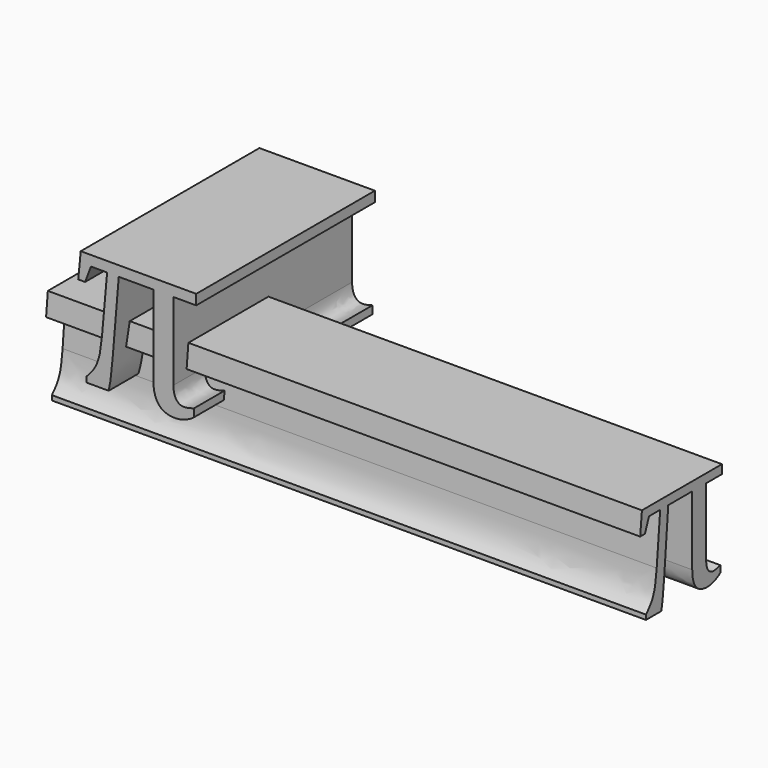
from build123d import *

# Parameters (mm, degrees)
F0_TEXT_SIZE = 28.1909998092
F1_DEPTH     = 25.4
F2_TEXT_SIZE = 24.4161502148
F3_DEPTH     = 67.564


# Not quite as in the source:
# - Text() gives the source's letters only with a copy of the font that has no kerning and outlines rounded to 1/6400 em; it was checked with that copy


with BuildPart() as f1:
    # F0 (on Front) → F1 (new body)
    with BuildSketch(Plane.XZ):
        with Locations((-62.7991110086, 28.3924750984)):
            Text('π', F0_TEXT_SIZE, font='Tinos', text_align=(TextAlign.LEFT, TextAlign.BOTTOM))
    extrude(amount=F1_DEPTH)

    # F2 (on Right) → F3 (join)
    with BuildSketch(Plane.YZ):
        with Locations((-23.8641817123, 23.5210377723)):
            Text('π', F2_TEXT_SIZE, font='Tinos', text_align=(TextAlign.LEFT, TextAlign.BOTTOM))
    extrude(amount=-F3_DEPTH)


solid = f1.part
